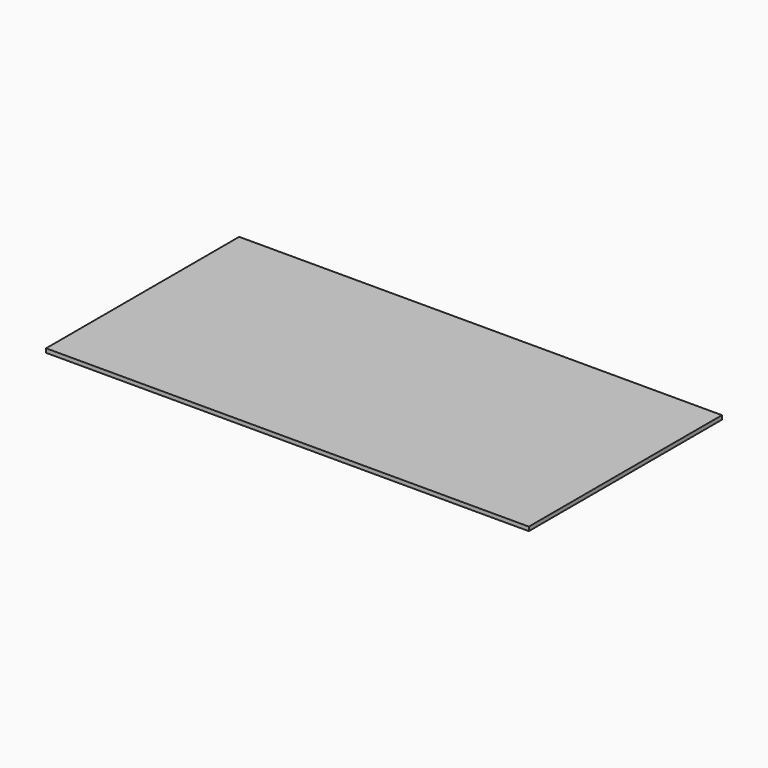
from build123d import *

# Parameters (mm, degrees)
F0_W     = 1524
F0_H     = 762
F1_DEPTH = 12.7


# Not quite as in the source:
# - a length typed as a fraction of an inch, garbled in the dataset ("3 / 203.2 mm" for 3/8 in), is restored


with BuildPart() as f1:
    # F0 (on Top) → F1 (new body)
    with BuildSketch(Plane.XY):
        Rectangle(F0_W, F0_H)
    extrude(amount=F1_DEPTH)


solid = f1.part
